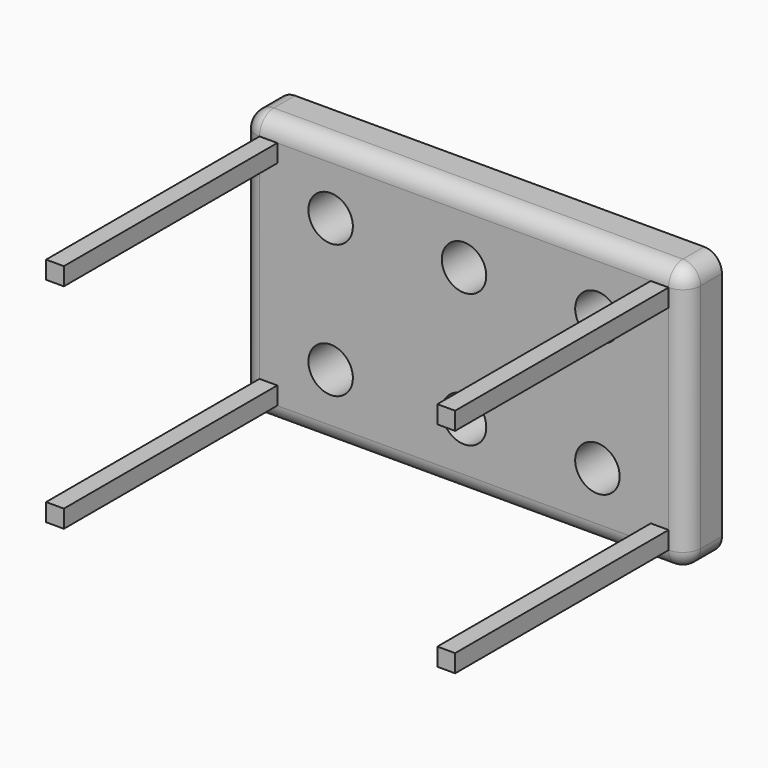
from build123d import *

# Parameters (mm, degrees)
F0_W         = 127
F0_H         = 76.2
F0_R         = 6.35
F1_DEPTH     = 12.7
F2_R         = 5.08
F3_T1_DEPTH  = 20.32
F3_S5_W      = 5.08
F3_S5_H      = 5.08
F3_T6_DEPTH  = 5.08
F3_S11_W     = 5.08
F3_S11_H     = 5.08
F3_T12_DEPTH = 5.08
F3_S17_W     = 5.08
F3_S17_H     = 5.08
F3_T18_DEPTH = 5.08
F3_S23_W     = 5.08
F3_S23_H     = 5.08
F3_T24_DEPTH = 5.08
F4_W         = 5.08
F4_H         = 5.08
F5_DEPTH     = 76.2


# Not quite as in the source:
# - a fillet or chamfer that OpenCascade refuses, or shapes differently, is made with other operations: its cross-section is extruded or revolved along the edge and cut away or added


with BuildPart() as f1:
    # F0 (on Front) → F1 (new body)
    with BuildSketch(Plane.XZ):
        with Locations((-0.4540607333, -4.4948741291)):
            Rectangle(F0_W, F0_H)
        with Locations((-38.5540607333, -23.5448741291)):
            Circle(F0_R, mode=Mode.SUBTRACT)
        with Locations((-0.4540607333, -23.5448741291)):
            Circle(F0_R, mode=Mode.SUBTRACT)
        with Locations((37.6459392667, -23.5448741291)):
            Circle(F0_R, mode=Mode.SUBTRACT)
        with Locations((-38.5540607333, 14.5551258709)):
            Circle(F0_R, mode=Mode.SUBTRACT)
        with Locations((-0.4540607333, 14.5551258709)):
            Circle(F0_R, mode=Mode.SUBTRACT)
        with Locations((37.6459392667, 14.5551258709)):
            Circle(F0_R, mode=Mode.SUBTRACT)
    extrude(amount=F1_DEPTH)

    # F2
    f2_edges = [f1.edges().sort_by_distance(p)[0] for p in [
        (-0.454061, -12.7, 33.605126),
        (-63.954061, -12.7, -4.494874),
        (-0.454061, -12.7, -42.594874),
        (63.045939, -12.7, -4.494874),
    ]]
    fillet(f2_edges, radius=F2_R)

    # F3: fillet of radius 5.08 on 4 edges, made by hand

    # F3_s2 → F3_t1 (cut)
    with BuildSketch(Plane.XZ.offset(-12.7)):
        with BuildLine():
            ThreePointArc((-63.9540607333, -37.5148741291), (-62.4661631817, -41.1069765775), (-58.8740607333, -42.5948741291))
            Line((-58.8740607333, -42.5948741291), (-63.9540607333, -42.5948741291))
            Line((-63.9540607333, -42.5948741291), (-63.9540607333, -37.5148741291))
        make_face()
        with BuildLine():
            ThreePointArc((63.0459392667, -37.5148741291), (61.5580417151, -41.1069765775), (57.9659392667, -42.5948741291))
            Line((57.9659392667, -42.5948741291), (63.0459392667, -42.5948741291))
            Line((63.0459392667, -42.5948741291), (63.0459392667, -37.5148741291))
        make_face()
        with BuildLine():
            ThreePointArc((57.9659392667, 33.6051258709), (61.5580417151, 32.1172283193), (63.0459392667, 28.5251258709))
            Line((63.0459392667, 28.5251258709), (63.0459392667, 33.6051258709))
            Line((63.0459392667, 33.6051258709), (57.9659392667, 33.6051258709))
        make_face()
        with BuildLine():
            ThreePointArc((-58.8740607333, 33.6051258709), (-62.4661631817, 32.1172283193), (-63.9540607333, 28.5251258709))
            Line((-63.9540607333, 28.5251258709), (-63.9540607333, 33.6051258709))
            Line((-63.9540607333, 33.6051258709), (-58.8740607333, 33.6051258709))
        make_face()
    extrude(amount=F3_T1_DEPTH, mode=Mode.SUBTRACT)


with BuildPart() as f3_tool4:
    # F3_s5 → F3_t6 (new body)
    with BuildSketch(Plane.XY.offset(28.5251258709)):
        with Locations((-61.4140607333, -10.16)):
            Rectangle(F3_S5_W, F3_S5_H)
    extrude(amount=F3_T6_DEPTH)

    # F3_s7 → F3_t8 (revolve, cut)
    with BuildSketch(Plane(origin=(-58.8740607333, -7.62, 28.5251258709), x_dir=(0.7071067812, 0.7071067812, 0), z_dir=(0.7071067812, -0.7071067812, 0))):
        with BuildLine():
            ThreePointArc((0, -5.08), (5.08, 0), (0, 5.08))
            Line((0, 5.08), (0, -5.08))
        make_face()
    revolve(axis=Axis((-58.8740607333, -7.62, 28.5251258709), (0, 0, 1)), mode=Mode.SUBTRACT)


with BuildPart() as f1_1:
    add(f1.part)

    # F3_t3: cut F3_tool4
    add(f3_tool4.part, mode=Mode.SUBTRACT)


with BuildPart() as f3_tool10:
    # F3_s11 → F3_t12 (new body)
    with BuildSketch(Plane.XY.offset(28.5251258709)):
        with Locations((60.5059392667, -10.16)):
            Rectangle(F3_S11_W, F3_S11_H)
    extrude(amount=F3_T12_DEPTH)

    # F3_s13 → F3_t14 (revolve, cut)
    with BuildSketch(Plane(origin=(57.9659392667, -7.62, 28.5251258709), x_dir=(-0.7071067812, 0.7071067812, 0), z_dir=(0.7071067812, 0.7071067812, 0))):
        with BuildLine():
            ThreePointArc((0, -5.08), (5.08, 0), (0, 5.08))
            Line((0, 5.08), (0, -5.08))
        make_face()
    revolve(axis=Axis((57.9659392667, -7.62, 28.5251258709), (0, 0, 1)), mode=Mode.SUBTRACT)


with BuildPart() as f1_2:
    add(f1_1.part)

    # F3_t9: cut F3_tool10
    add(f3_tool10.part, mode=Mode.SUBTRACT)


with BuildPart() as f3_tool16:
    # F3_s17 → F3_t18 (new body)
    with BuildSketch(Plane.YZ.offset(57.9659392667)):
        with Locations((-10.16, -40.0548741291)):
            Rectangle(F3_S17_W, F3_S17_H)
    extrude(amount=F3_T18_DEPTH)

    # F3_s19 → F3_t20 (revolve, cut)
    with BuildSketch(Plane(origin=(57.9659392667, -7.62, -37.5148741291), x_dir=(0, 0.7071067812, 0.7071067812), z_dir=(0, 0.7071067812, -0.7071067812))):
        with BuildLine():
            ThreePointArc((0, -5.08), (5.08, 0), (0, 5.08))
            Line((0, 5.08), (0, -5.08))
        make_face()
    revolve(axis=Axis((57.9659392667, -7.62, -37.5148741291), (1, 0, 0)), mode=Mode.SUBTRACT)


with BuildPart() as f1_3:
    add(f1_2.part)

    # F3_t15: cut F3_tool16
    add(f3_tool16.part, mode=Mode.SUBTRACT)


with BuildPart() as f3_tool22:
    # F3_s23 → F3_t24 (new body)
    with BuildSketch(Plane.YZ.offset(-58.8740607333)):
        with Locations((-10.16, -40.0548741291)):
            Rectangle(F3_S23_W, F3_S23_H)
    extrude(amount=-F3_T24_DEPTH)

    # F3_s25 → F3_t26 (revolve, cut)
    with BuildSketch(Plane(origin=(-58.8740607333, -7.62, -37.5148741291), x_dir=(0, 0.7071067812, 0.7071067812), z_dir=(0, -0.7071067812, 0.7071067812))):
        with BuildLine():
            ThreePointArc((0, -5.08), (5.08, 0), (0, 5.08))
            Line((0, 5.08), (0, -5.08))
        make_face()
    revolve(axis=Axis((-58.8740607333, -7.62, -37.5148741291), (-1, 0, 0)), mode=Mode.SUBTRACT)


with BuildPart() as f1_4:
    add(f1_3.part)

    # F3_t21: cut F3_tool22
    add(f3_tool22.part, mode=Mode.SUBTRACT)

    # F4 (on face) → F5 (join)
    with BuildSketch(Plane.XZ.offset(12.7)):
        with Locations((-56.3340607333, -34.9748741291)):
            Rectangle(F4_W, F4_H)
        with Locations((55.4259392667, -34.9748741291)):
            Rectangle(F4_W, F4_H)
        with Locations((55.4259392667, 25.9851258709)):
            Rectangle(F4_W, F4_H)
        with Locations((-56.3340607333, 25.9851258709)):
            Rectangle(F4_W, F4_H)
    extrude(amount=F5_DEPTH)


solid = f1_4.part
